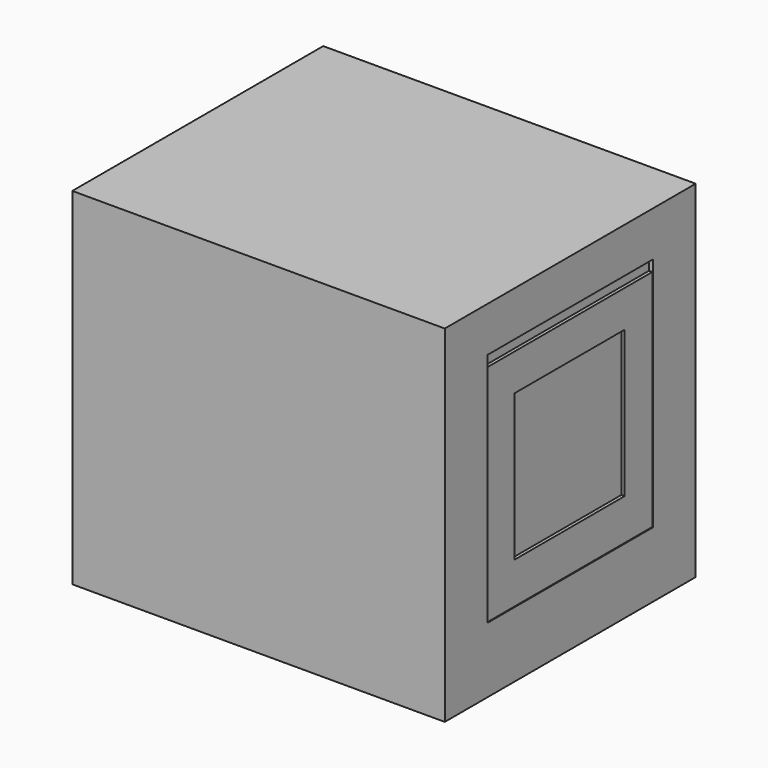
from build123d import *

# Parameters (mm, degrees)
F0_W     = 265
F0_H     = 286
F1_DEPTH = 455
F2_W     = 168.7
F2_H     = 179.4
F3_DEPTH = 5
F4_W     = 384
F4_H     = 424
F5_DEPTH = 456
F6_W     = 253.7
F6_H     = 288.8
F7_DEPTH = 5


with BuildPart() as f1:
    # F0 (on Right) → F1 (new body)
    with BuildSketch(Plane.YZ):
        Rectangle(F0_W, F0_H)
    extrude(amount=F1_DEPTH)

    # F2 (on face) → F3 (cut)
    with BuildSketch(Plane.YZ.offset(455)):
        with Locations((0, 8.3)):
            Rectangle(F2_W, F2_H)
    extrude(amount=-F3_DEPTH, mode=Mode.SUBTRACT)


with BuildPart() as f5:
    # F4 (on Right) → F5 (new body)
    with BuildSketch(Plane.YZ):
        Rectangle(F4_W, F4_H)
    extrude(amount=F5_DEPTH)

    # F6 (on face) → F7 (cut)
    with BuildSketch(Plane.YZ.offset(456)):
        with Locations((0, 12.6)):
            Rectangle(F6_W, F6_H)
    extrude(amount=-F7_DEPTH, mode=Mode.SUBTRACT)


solid = Compound([f1.part, f5.part])
